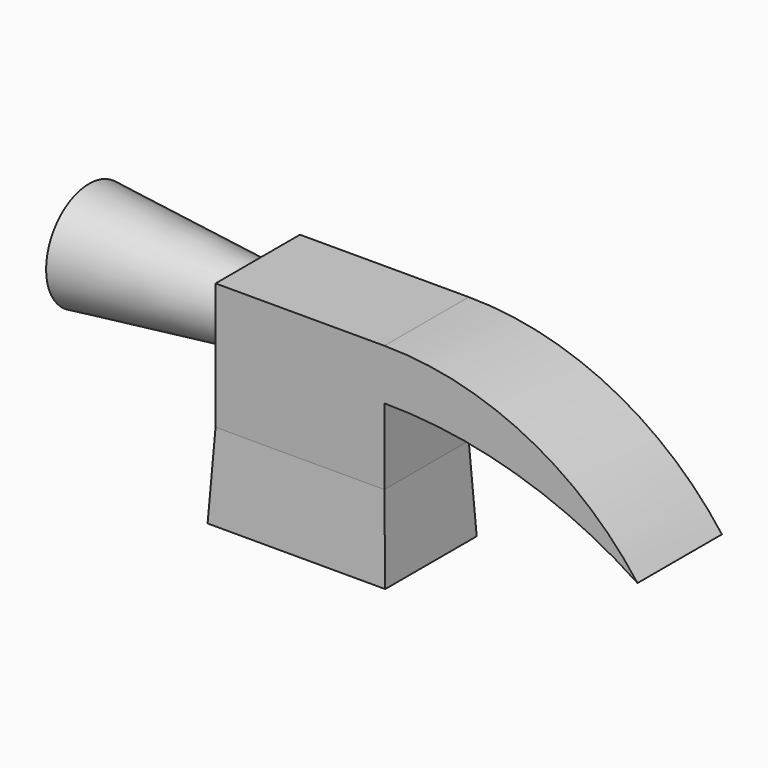
from build123d import *

# Parameters (mm, degrees)
F0_W       = 40
F0_H       = 29.999999
F1_DEPTH   = 12.5
F2_R       = 8.5
F3_DEPTH   = 40
F3_TAPER   = -6
F5_DEPTH   = 12.5
F1_FACE1_W = 40
F1_FACE1_H = 25
F6_DEPTH   = 20
F6_TAPER   = -3


with BuildPart() as f1:
    # F0 (on Front) → F1 (new body, symmetric)
    with BuildSketch(Plane.XZ):
        with Locations((0, 14.999999)):
            Rectangle(F0_W, F0_H)
    extrude(amount=F1_DEPTH, both=True)

    # F2 (on face) → F3 (join)
    with BuildSketch(Plane(origin=(-20, 0, 0), x_dir=(0, -1, 0), z_dir=(-1, 0, 0))):
        with Locations((0, 20)):
            Circle(F2_R)
    extrude(amount=F3_DEPTH, taper=F3_TAPER)

    # F4 (on Front) → F5 (join, symmetric)
    with BuildSketch(Plane.XZ):
        with BuildLine():
            ThreePointArc((20, 18), (51.32092, 13.403065), (80, 0))
            ThreePointArc((80, 0), (53.54102, 22.082039), (20, 30))
            Line((20, 30), (20, 18))
        make_face()
    extrude(amount=F5_DEPTH, both=True)


with BuildPart() as f6:
    # F1_face1 (on face) → F6 (new body)
    with BuildSketch(Plane(origin=(0, 0, 0), x_dir=(1, 0, 0), z_dir=(0, 0, -1))):
        Rectangle(F1_FACE1_W, F1_FACE1_H)
    extrude(amount=F6_DEPTH, taper=F6_TAPER)


solid = Compound([f1.part, f6.part])
